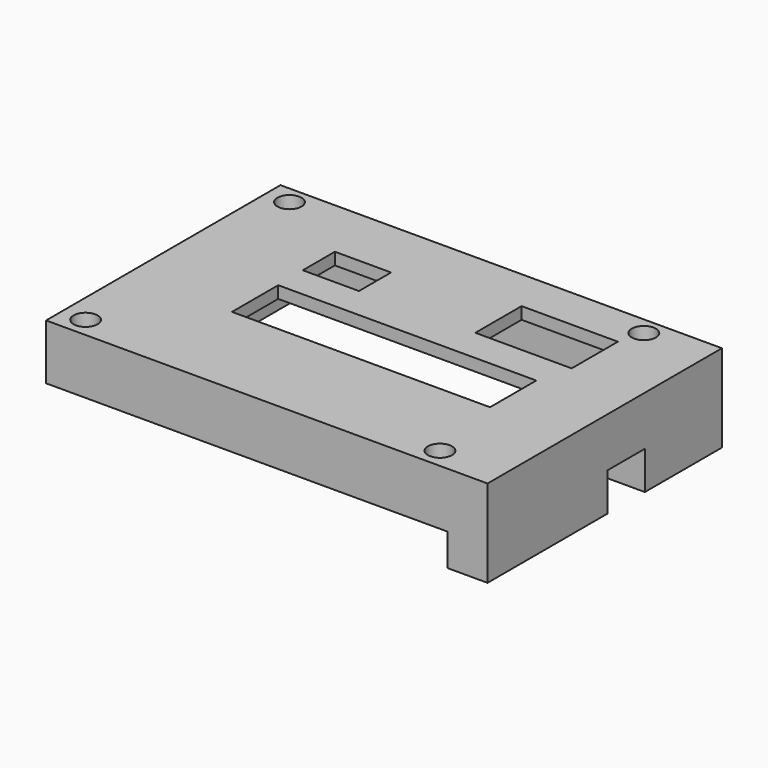
from build123d import *

# Parameters (mm, degrees)
F0_W      = 110
F0_H      = 73
F1_DEPTH  = 13.8
F2_W      = 84
F2_H      = 54
F3_DEPTH  = 10.8
F4_W      = 10
F4_H      = 73
F5_DEPTH  = 8
F6_R      = 1.75
F7_DEPTH  = 25
F8_R      = 3
F9_DEPTH  = 5
F10_W     = 64.3
F10_H     = 14.4
F10_W_2   = 24
F10_W_3   = 14
F10_H_2   = 10
F11_DEPTH = 25
F12_W     = 11.6
F12_H     = 9.5
F13_DEPTH = 25
F15_START = -27.4
F15_DEPTH = 10


# Not quite as in the source:
# - a pattern or mirror of a feature is missing from the dataset's text; its kind, count and spacing are read off the source's solid


with BuildPart() as f1:
    # F0 (on Top) → F1 (new body)
    with BuildSketch(Plane.XY):
        with Locations((55, 36.5)):
            Rectangle(F0_W, F0_H)
    extrude(amount=F1_DEPTH)

    # F2 (on face) → F3 (cut)
    with BuildSketch(Plane(origin=(0, 0, 0), x_dir=(1, 0, 0), z_dir=(0, 0, -1))):
        with Locations((58, -37)):
            Rectangle(F2_W, F2_H)
    extrude(amount=-F3_DEPTH, mode=Mode.SUBTRACT)

    # F4 (on face) → F5 (join)
    with BuildSketch(Plane(origin=(0, 0, 0), x_dir=(1, 0, 0), z_dir=(0, 0, -1))):
        with Locations((105, -36.5)):
            Rectangle(F4_W, F4_H)
    extrude(amount=F5_DEPTH)

    # F6 (on face) → F7 (cut)
    with BuildSketch(Plane.XY.offset(13.8)):
        with Locations((5.85, 5)):
            Circle(F6_R)
        with Locations((94.15, 5)):
            Circle(F6_R)
        with Locations((94.15, 68.5)):
            Circle(F6_R)
        with Locations((5.85, 68.5)):
            Circle(F6_R)
    extrude(amount=-F7_DEPTH, mode=Mode.SUBTRACT)

    # F8 (on face) → F9 (cut)
    with BuildSketch(Plane.XY.offset(13.8)):
        with Locations((5.85, 68.5)):
            Circle(F8_R)
        with Locations((5.85, 5)):
            Circle(F8_R)
        with Locations((94.15, 5)):
            Circle(F8_R)
        with Locations((94.15, 68.5)):
            Circle(F8_R)
    extrude(amount=-F9_DEPTH, mode=Mode.SUBTRACT)

    # F10 (on face) → F11 (cut)
    with BuildSketch(Plane.XY.offset(13.8)):
        with Locations((58.15, 32.6)):
            Rectangle(F10_W, F10_H)
        with Locations((80.48, 55.3)):
            Rectangle(F10_W_2, F10_H)
        with Locations((32.8, 52.7)):
            Rectangle(F10_W_3, F10_H_2)
    extrude(amount=-F11_DEPTH, mode=Mode.SUBTRACT)

    # F12 (on face) → F13 (cut)
    with BuildSketch(Plane.YZ.offset(110)):
        with Locations((43.2, -3.25)):
            Rectangle(F12_W, F12_H)
    extrude(amount=-F13_DEPTH, mode=Mode.SUBTRACT)

    # F14 (on face) → F15 (join)
    with BuildSketch(Plane.XZ.offset(F15_START)):
        Polygon((94, -8), (97.5, -8), (97.5, 2), (100, 2), (100, 4.5), (100, 13.8), (96, 13.8), (96, 4.5), (94, -1.75), align=None)
    f15 = extrude(amount=-F15_DEPTH)

    # F15_copies: F15 across plane
    add(f15.mirror(Plane.ZX.offset(43.2)))


solid = f1.part
